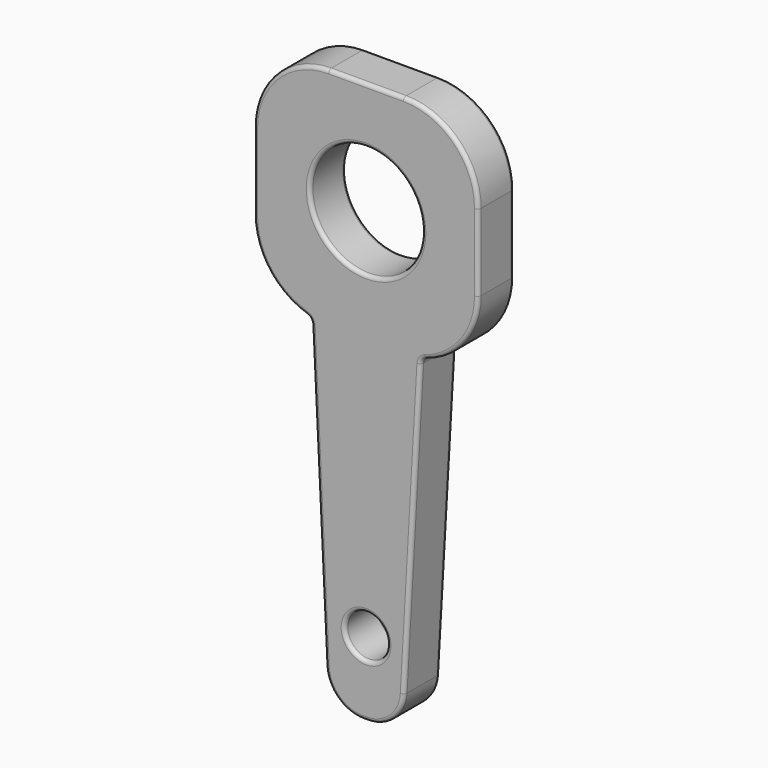
from build123d import *

# Parameters (mm, degrees)
F0_R         = 28.25
F0_R_2       = 75
F1_DEPTH     = 60
F3_T1_DEPTH  = 545.1617031196
F3_T3_DEPTH  = 546.1296912431
F3_T5_DEPTH  = 560
F4_R         = 10
F5_R         = 5
F6_T1_DEPTH  = 60
F6_T4_ANGLE  = 87.2619735231
F6_T6_ANGLE  = 87.2619735231
F6_T8_ANGLE  = 86.7878998104
F6_T10_ANGLE = 86.7878998104


# Not quite as in the source:
# - a fillet or chamfer that OpenCascade refuses, or shapes differently, is made with other operations: its cross-section is extruded or revolved along the edge and cut away or added
# - a feature of the source that left no trace in its solid (it failed there, or was rolled back) is left out


with BuildPart() as f1:
    # F0 (on Front) → F1 (new body)
    with BuildSketch(Plane.XZ):
        Polygon((-73.3905308122, 30.889634043), (-51.8618531352, -419.2752103038), (48.1381468648, -419.2752103038), (73.3907752815, 30.6960952328), (150, 30.889634043), (150, 330.889634043), (-150, 330.889634043), (-150, 30.889634043), align=None)
        with Locations((0, -320.0415968895)):
            Circle(F0_R, mode=Mode.SUBTRACT)
        with Locations((0, 180.889634043)):
            Circle(F0_R_2, mode=Mode.SUBTRACT)
    extrude(amount=F1_DEPTH)

    # F3: fillet of radius 100 on 4 edges, made by hand

    # F3_s2 → F3_t1 (cut)
    with BuildSketch(Plane.XZ.offset(-242.5808515598)):
        with BuildLine():
            ThreePointArc((73.3907752815, 30.6960952328), (128.5464115289, 66.0312545554), (150, 127.9219746669))
            Line((150, 127.9219746669), (150, 30.889634043))
            Line((150, 30.889634043), (73.3907752815, 30.6960952328))
        make_face()
    extrude(amount=F3_T1_DEPTH, mode=Mode.SUBTRACT)

    # F3_s4 → F3_t3 (cut)
    with BuildSketch(Plane.XZ.offset(-243.0648456216)):
        with BuildLine():
            ThreePointArc((-150, 128.1155722916), (-128.5463337184, 66.2247534297), (-73.3905308122, 30.889634043))
            Line((-73.3905308122, 30.889634043), (-150, 30.889634043))
            Line((-150, 30.889634043), (-150, 128.1155722916))
        make_face()
    extrude(amount=F3_T3_DEPTH, mode=Mode.SUBTRACT)

    # F3_s6 → F3_t5 (cut)
    with BuildSketch(Plane.XZ.offset(-250)):
        with BuildLine():
            ThreePointArc((150, 230.889634043), (120.7106781187, 301.6003121616), (50, 330.889634043))
            Line((50, 330.889634043), (150, 330.889634043))
            Line((150, 330.889634043), (150, 230.889634043))
        make_face()
        with BuildLine():
            ThreePointArc((-50, 330.889634043), (-120.7106781187, 301.6003121616), (-150, 230.889634043))
            Line((-150, 230.889634043), (-150, 330.889634043))
            Line((-150, 330.889634043), (-50, 330.889634043))
        make_face()
    extrude(amount=F3_T5_DEPTH, mode=Mode.SUBTRACT)

    # F4
    f4_edges = [f1.edges().sort_by_distance(p)[0] for p in [
        (-73.390531, -30, 30.889634),
        (73.390775, -30, 30.696095),
    ]]
    fillet(f4_edges, radius=F4_R)

    # F5
    f5_edges = [f1.edges().sort_by_distance(p)[0] for p in [
        (-130.632125, 0, 68.967788),
        (-75.114274, 0, 29.298651),
        (-150, 0, 179.502603),
        (-62.453571, 0, -197.802299),
        (-120.710678, 0, 301.600312),
        (-1.861853, 0, -419.27521),
        (0, 0, 330.889634),
        (60.563678, 0, -197.867278),
        (120.710678, 0, 301.600312),
        (75.080994, 0, 29.121046),
        (150, 0, 179.405804),
        (130.615106, 0, 68.750997),
        (-28.25, 0, -320.041597),
        (-75, 0, 180.889634),
        (-130.632125, -60, 68.967788),
        (-75.114274, -60, 29.298651),
        (-150, -60, 179.502603),
        (-62.453571, -60, -197.802299),
        (-120.710678, -60, 301.600312),
        (-1.861853, -60, -419.27521),
        (0, -60, 330.889634),
        (60.563678, -60, -197.867278),
        (120.710678, -60, 301.600312),
        (75.080994, -60, 29.121046),
        (150, -60, 179.405804),
        (130.615106, -60, 68.750997),
        (-28.25, -60, -320.041597),
        (-75, -60, 180.889634),
    ]]
    fillet(f5_edges, radius=F5_R)

    # F6: fillet of radius 50 on 2 edges, made by hand

    # F6_s2 → F6_t1 (cut)
    with BuildSketch(Plane.XZ):
        with BuildLine():
            ThreePointArc((0.8654974445, -419.2752103038), (35.2160366942, -405.6075712682), (50.7869450983, -372.0768284339))
            Line((50.7869450983, -372.0768284339), (48.1381468648, -419.2752103038))
            Line((48.1381468648, -419.2752103038), (0.8654974445, -419.2752103038))
        make_face()
        with BuildLine():
            ThreePointArc((-54.1388263505, -371.6636798405), (-38.6964613108, -405.4651500442), (-4.1959067996, -419.2752103038))
            Line((-4.1959067996, -419.2752103038), (-51.8618531352, -419.2752103038))
            Line((-51.8618531352, -419.2752103038), (-54.1388263505, -371.6636798405))
        make_face()
    extrude(amount=F6_T1_DEPTH, mode=Mode.SUBTRACT)

    # F6_s3 → F6_t4 (revolve, cut)
    with BuildSketch(Plane.YZ.offset(-4.1959067996)):
        with BuildLine():
            ThreePointArc((0, -414.2752103038), (-1.4644660941, -417.8107442097), (-5, -419.2752103038))
            Line((-5, -419.2752103038), (0, -419.2752103038))
            Line((0, -419.2752103038), (0, -414.2752103038))
        make_face()
    revolve(axis=Axis((-4.1959067996, 0, -369.2752103038), (0, 1, 0)), revolution_arc=F6_T4_ANGLE, mode=Mode.SUBTRACT)

    # F6_s5 → F6_t6 (revolve, cut)
    with BuildSketch(Plane(origin=(17.6103390671, 0, -368.2323486843), x_dir=(0, 1, 0), z_dir=(-0.0477693907, 0, 0.998858391))):
        with BuildLine():
            ThreePointArc((-60, 66.8311685248), (-58.5355339059, 70.3667024307), (-55, 71.8311685248))
            Line((-55, 71.8311685248), (-60, 71.8311685248))
            Line((-60, 71.8311685248), (-60, 66.8311685248))
        make_face()
    revolve(axis=Axis((-4.1959067996, -60, -369.2752103038), (0, -1, 0)), revolution_arc=F6_T6_ANGLE, mode=Mode.SUBTRACT)

    # F6_s7 → F6_t8 (revolve, cut)
    with BuildSketch(Plane(origin=(-20.6561380445, 0, -368.067404701), x_dir=(0, 1, 0), z_dir=(0.0560323626, 0, 0.9984289531))):
        with BuildLine():
            ThreePointArc((0, -66.5555001912), (-1.4644660941, -70.0910340971), (-5, -71.5555001912))
            Line((-5, -71.5555001912), (0, -71.5555001912))
            Line((0, -71.5555001912), (0, -66.5555001912))
        make_face()
    revolve(axis=Axis((0.8654974445, 0, -369.2752103038), (0, 1, 0)), revolution_arc=F6_T8_ANGLE, mode=Mode.SUBTRACT)

    # F6_s9 → F6_t10 (revolve, cut)
    with BuildSketch(Plane.YZ.offset(0.8654974445)):
        with BuildLine():
            ThreePointArc((-60, -414.2752103038), (-58.5355339059, -417.8107442097), (-55, -419.2752103038))
            Line((-55, -419.2752103038), (-60, -419.2752103038))
            Line((-60, -419.2752103038), (-60, -414.2752103038))
        make_face()
    revolve(axis=Axis((0.8654974445, -60, -369.2752103038), (0, -1, 0)), revolution_arc=F6_T10_ANGLE, mode=Mode.SUBTRACT)


solid = f1.part
